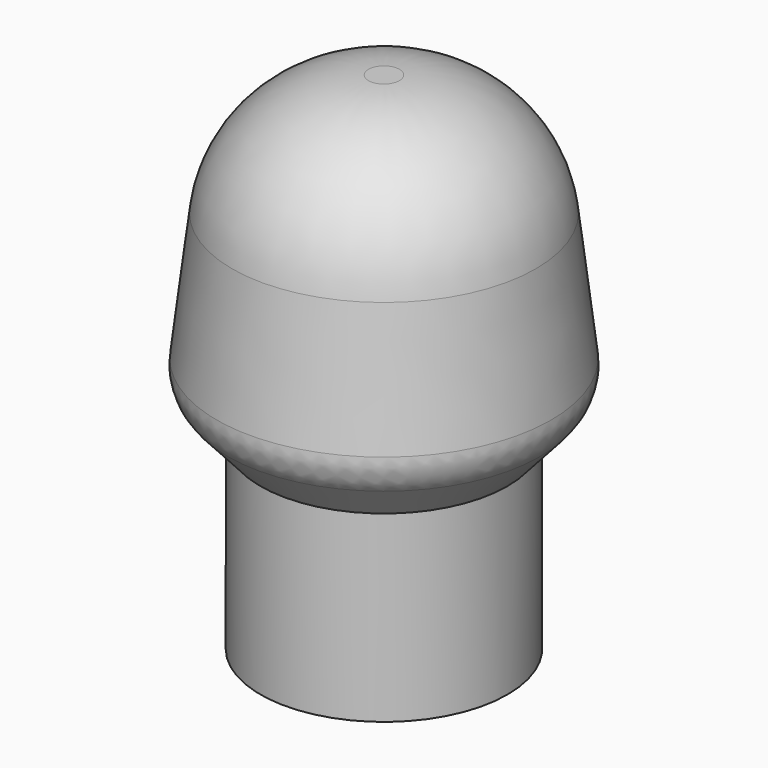
from build123d import *

# Parameters (mm, degrees)
F0_R        = 6.85
F1_DEPTH    = 8
F4_R        = 7.62
F5_S5_R     = 6.85
F5_T6_DEPTH = 16
F6_R        = 2.54


# Not quite as in the source:
# - a fillet or chamfer that OpenCascade refuses, or shapes differently, is made with other operations: its cross-section is extruded or revolved along the edge and cut away or added


with BuildPart() as f1:
    # F0 (on Top) → F1 (new body)
    with BuildSketch(Plane.XY):
        Circle(F0_R)
    extrude(amount=-F1_DEPTH)

    # F2 (on Front) → F3 (revolve)
    with BuildSketch(Plane.XZ):
        Polygon((-10.0059127435, 0), (0, 0), (0, 20), (-7.62, 20), align=None)
    revolve(axis=Axis((0, 0, 10), (0, 0, 1)))

    # F4
    f4_edges = [f1.edges().sort_by_distance(p)[0] for p in [
        (7.62, 0, 20),
    ]]
    fillet(f4_edges, radius=F4_R)

    # F5: chamfer of 5.08 on 1 edges, made by hand


with BuildPart() as f5_tool2:
    # F5_s3 → F5_t4 (revolve)
    with BuildSketch(Plane.XZ):
        Polygon((-9.4041577027, 5.0442334275), (-4.9259127435, 0), (-10.0059127435, 0), align=None)
    revolve(axis=Axis((0, 0, 0), (0, 0, 1)))

    # F5_s5 → F5_t6 (cut, symmetric)
    with BuildSketch(Plane.XY.offset(2.5)):
        Circle(F5_S5_R)
    extrude(amount=F5_T6_DEPTH, both=True, mode=Mode.SUBTRACT)


with BuildPart() as f1_1:
    add(f1.part)

    # F5_t1: cut F5_tool2
    add(f5_tool2.part, mode=Mode.SUBTRACT)

    # F6
    f6_edges = [f1_1.edges().sort_by_distance(p)[0] for p in [
        (9.404158, 0, 5.044233),
    ]]
    fillet(f6_edges, radius=F6_R)


solid = f1_1.part
